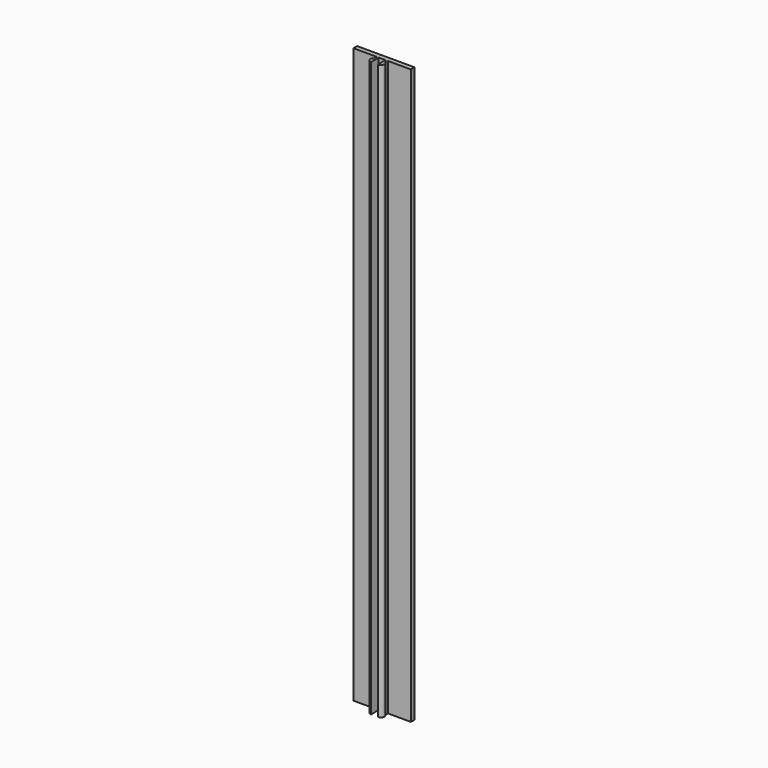
from build123d import *

# Parameters (mm, degrees)
F1_DEPTH    = 200
F2_T1_DEPTH = 203.7080992435
F3_T1_DEPTH = 206.4966679694


# Not quite as in the source:
# - a fillet or chamfer that OpenCascade refuses, or shapes differently, is made with other operations: its cross-section is extruded or revolved along the edge and cut away or added


with BuildPart() as f1:
    # F0 (on Top) → F1 (new body)
    with BuildSketch(Plane.XY):
        Polygon((-10, 4.9), (-10, 3.3), (-2, 3.3), (-2, 2), (-2.5, 2), (-2.5, 0.8), (-2.5, 0), (-1.2, 0), (-1.2, 0.8), (-1.2, 3.3), (1.2, 3.3), (1.2, 0.8), (1.2, 0), (2.5, 0), (2.5, 0.8), (2.5, 2), (2, 2), (2, 3.3), (10, 3.3), (10, 4.9), align=None)
    extrude(amount=F1_DEPTH)

    # F2: fillet of radius 0.8 on 2 edges, made by hand

    # F2_s2 → F2_t1 (cut)
    with BuildSketch(Plane.XY.offset(-1.8540496218)):
        with BuildLine():
            ThreePointArc((2, 2), (2.3633249581, 1.7055937468), (2.5, 1.2583801513))
            Line((2.5, 1.2583801513), (2.5, 2))
            Line((2.5, 2), (2, 2))
        make_face()
        with BuildLine():
            ThreePointArc((-2.5, 1.2583801513), (-2.3633249581, 1.7055937468), (-2, 2))
            Line((-2, 2), (-2.5, 2))
            Line((-2.5, 2), (-2.5, 1.2583801513))
        make_face()
    extrude(amount=F2_T1_DEPTH, mode=Mode.SUBTRACT)

    # F3: fillet of radius 1.3 on 2 edges, made by hand

    # F3_s2 → F3_t1 (cut)
    with BuildSketch(Plane.XY.offset(-3.2483339847)):
        with BuildLine():
            ThreePointArc((-1.2006664061, 0), (-2.1050706843, 0.3661622723), (-2.5, 1.2583801513))
            Line((-2.5, 1.2583801513), (-2.5259866719, 1.2575477543))
            ThreePointArc((-2.5259866719, 1.2575477543), (-2.526, 0.6291900756), (-2.526, 0))
            Line((-2.526, 0), (-2.5, -0.026))
            Line((-2.5, -0.026), (-1.2006664061, -0.026))
            Line((-1.2006664061, -0.026), (-1.2006664061, 0))
        make_face()
        with BuildLine():
            ThreePointArc((2.5, 1.2583801513), (2.1050706843, 0.3661622723), (1.2006664061, 0))
            Line((1.2006664061, 0), (1.2006664061, -0.026))
            Line((1.2006664061, -0.026), (2.5, -0.026))
            Line((2.5, -0.026), (2.526, 0))
            ThreePointArc((2.526, 0), (2.526, 0.6291900756), (2.5259866719, 1.2575477543))
            Line((2.5259866719, 1.2575477543), (2.5, 1.2583801513))
        make_face()
    extrude(amount=F3_T1_DEPTH, mode=Mode.SUBTRACT)


solid = f1.part
